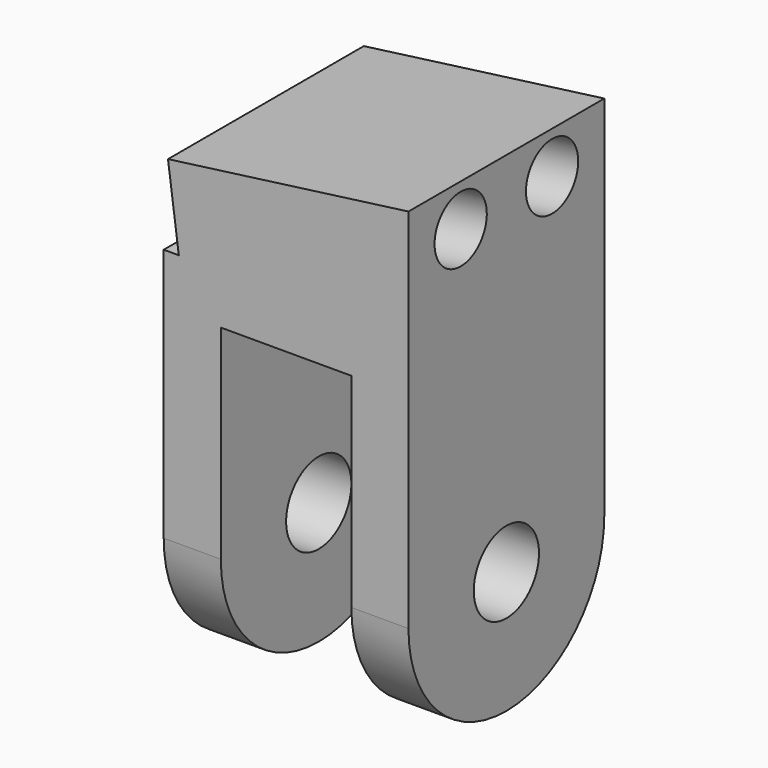
from build123d import *

# Parameters (mm, degrees)
F0_W     = 15
F0_H     = 30
F1_DEPTH = 15
F2_W     = 8
F2_H     = 20
F3_DEPTH = 25.4
F4_R     = 7.49999
F5_R     = 2
F6_DEPTH = 25.4
F7_R     = 2.5
F8_DEPTH = 25.4


# Not quite as in the source:
# - a fillet or chamfer is up to 0.001 mm smaller than in the source, because OpenCascade refuses the exact size


with BuildPart() as f1:
    # F0 (on Front) → F1 (new body)
    with BuildSketch(Plane.XZ):
        Rectangle(F0_W, F0_H)
    extrude(amount=F1_DEPTH)

    # F2 (on face) → F3 (cut)
    with BuildSketch(Plane.XZ.offset(15)):
        with Locations((0, -5)):
            Rectangle(F2_W, F2_H)
        Polygon((-7.5, 15), (-7.5, 13), (-7.2379912664, 13.0349344978), align=None)
        Polygon((-7.2379912664, 13.0349344978), (-7.5, 13), (-7.5, 8.0614046952), (-6.5748539594, 8.0614046952), align=None)
        Polygon((-7.5, 15), (-7.2379912664, 13.0349344978), (7.5, 15), align=None)
    extrude(amount=-F3_DEPTH, mode=Mode.SUBTRACT)

    # F4 (radius 7.5 in the source; OpenCascade refuses exactly that, so slightly less here)
    f4_edges = [f1.edges().sort_by_distance(p)[0] for p in [
        (-5.75, -15, -15),
        (-5.75, 0, -15),
        (5.75, 0, -15),
        (5.75, -15, -15),
    ]]
    fillet(f4_edges, radius=F4_R)

    # F5 (on face) → F6 (cut)
    with BuildSketch(Plane(origin=(-5.403930131, 0, -0.7205240175), x_dir=(0, -1, 0), z_dir=(-0.9912279007, 0, -0.1321637201))):
        with Locations((4, 11.3289700367)):
            Circle(F5_R)
        with Locations((11, 11.3289700367)):
            Circle(F5_R)
    extrude(amount=-F6_DEPTH, mode=Mode.SUBTRACT)

    # F7 (on face) → F8 (cut)
    with BuildSketch(Plane(origin=(-7.5, 0, 0), x_dir=(0, -1, 0), z_dir=(-1, 0, 0))):
        with Locations((7.5, -7.5)):
            Circle(F7_R)
    extrude(amount=-F8_DEPTH, mode=Mode.SUBTRACT)


solid = f1.part
